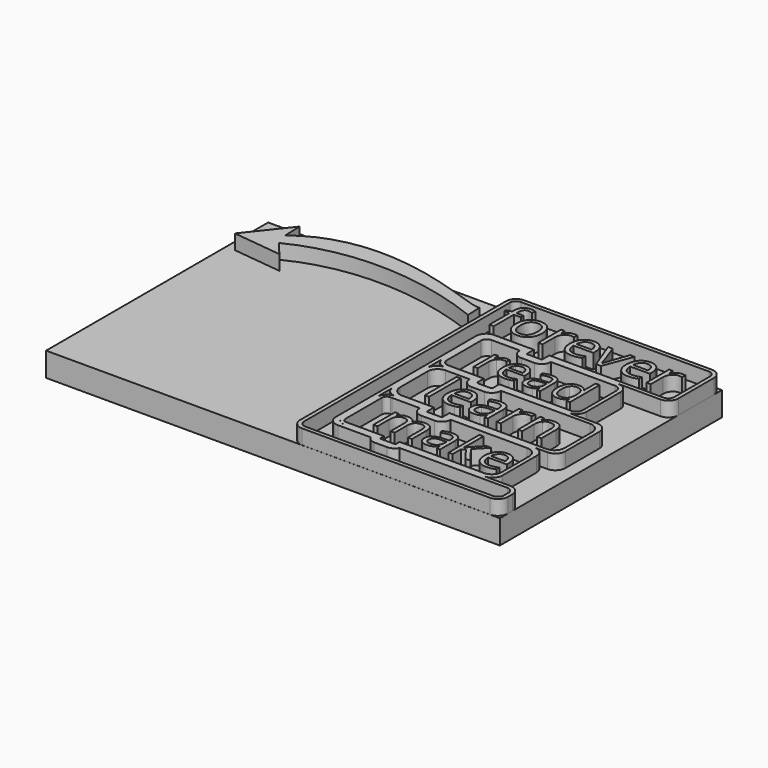
from build123d import *

# Parameters (mm, degrees)
F0_TEXT_SIZE   = 5.4091811762
F0_W           = 0.4318574544
F0_H           = 4.046479385
F1_DEPTH       = 1.5
F0_TEXT_SIZE_2 = 5.1478958792
F2_DEPTH       = 1.5
F3_DEPTH       = 1.5
F4_DEPTH       = 1.5
F5_W           = 28.2222777605
F5_H           = 2.4435883388
F6_DEPTH       = 21.1379435506
F7_DEPTH       = 25
F9_DEPTH       = 1.5


# Not quite as in the source:
# - ends of sketch curves that miss each other by under 0.0002 mm in the source are joined
# - Text() gives the source's letters only with a copy of the font that has no kerning and outlines rounded to 1/6400 em; it was checked with that copy


with BuildPart() as f1:
    # F0 (on Top) → F1 (new body)
    with BuildSketch(Plane.XY):
        with Locations((-20.2342048287, -5.0012101419)):
            Text('forever', F0_TEXT_SIZE, font='Open Sans', text_align=(TextAlign.LEFT, TextAlign.BOTTOM))
        with BuildLine():
            add(Edge.make_bspline(
                [(-14.8840140161, -8.7097081899), (-14.7069441142, -8.7097081899), (-14.5663754641, -8.7392198402)],
                knots=[0, 0, 0, 1, 1, 1], degree=2))
            add(Edge.make_bspline(
                [(-15.3429978406, -8.8506651512), (-15.1340864213, -8.7097081899), (-14.8840140161, -8.7097081899)],
                knots=[0, 0, 0, 1, 1, 1], degree=2))
            add(Edge.make_bspline(
                [(-15.6994675114, -9.2510139863), (-15.5519092599, -8.9916221126), (-15.3429978406, -8.8506651512)],
                knots=[0, 0, 0, 1, 1, 1], degree=2))
            Line((-15.6994675114, -9.2510139863), (-15.7188830708, -9.2510139863))
            Line((-15.7188830708, -9.2510139863), (-15.7654804134, -8.7586353996))
            Line((-15.7654804134, -8.7586353996), (-16.0978747905, -8.7586353996))
            Line((-16.0978747905, -8.7586353996), (-16.0978747905, -11.4185670391))
            Line((-16.0978747905, -11.4185670391), (-15.6948077771, -11.4185670391))
            Line((-15.6948077771, -11.4185670391), (-15.6948077771, -9.9911351111))
            add(Edge.make_bspline(
                [(-15.4657041761, -9.3383840037), (-15.6948077771, -9.6004940557), (-15.6948077771, -9.9911351111)],
                knots=[0, 0, 0, 1, 1, 1], degree=2))
            add(Edge.make_bspline(
                [(-14.9135256664, -9.0762739516), (-15.236600575, -9.0762739516), (-15.4657041761, -9.3383840037)],
                knots=[0, 0, 0, 1, 1, 1], degree=2))
            add(Edge.make_bspline(
                [(-14.6222922752, -9.1127752033), (-14.786936219, -9.0762739516), (-14.9135256664, -9.0762739516)],
                knots=[0, 0, 0, 1, 1, 1], degree=2))
            Line((-14.6222922752, -9.1127752033), (-14.5663754641, -8.7392198402))
        make_face()
        with BuildLine():
            add(Edge.make_bspline(
                [(-12.944787942, -11.4674942488), (-13.5342443258, -11.4674942488), (-13.8755698602, -11.1079180885)],
                knots=[0, 0, 0, 1, 1, 1], degree=2))
            add(Edge.make_bspline(
                [(-12.4850274951, -11.4271098852), (-12.6752999774, -11.4674942488), (-12.944787942, -11.4674942488)],
                knots=[0, 0, 0, 1, 1, 1], degree=2))
            add(Edge.make_bspline(
                [(-12.0811838594, -11.2950840812), (-12.2947550129, -11.3867255216), (-12.4850274951, -11.4271098852)],
                knots=[0, 0, 0, 1, 1, 1], degree=2))
            Line((-12.0811838594, -11.2950840812), (-12.0811838594, -10.9355079209))
            add(Edge.make_bspline(
                [(-12.9300321169, -11.1149076899), (-12.5005599427, -11.1149076899), (-12.0811838594, -10.9355079209)],
                knots=[0, 0, 0, 1, 1, 1], degree=2))
            add(Edge.make_bspline(
                [(-13.5622027313, -10.8722131972), (-13.3377588645, -11.1149076899), (-12.9300321169, -11.1149076899)],
                knots=[0, 0, 0, 1, 1, 1], degree=2))
            add(Edge.make_bspline(
                [(-13.7990725561, -10.1612154115), (-13.7866465981, -10.6295187046), (-13.5622027313, -10.8722131972)],
                knots=[0, 0, 0, 1, 1, 1], degree=2))
            Line((-13.7990725561, -10.1612154115), (-11.96702037, -10.1612154115))
            Line((-11.96702037, -10.1612154115), (-11.96702037, -9.9064832721))
            add(Edge.make_bspline(
                [(-12.2582537612, -9.0386077663), (-11.96702037, -9.3675073428), (-11.96702037, -9.9064832721)],
                knots=[0, 0, 0, 1, 1, 1], degree=2))
            add(Edge.make_bspline(
                [(-13.0488553405, -8.7097081899), (-12.5494871524, -8.7097081899), (-12.2582537612, -9.0386077663)],
                knots=[0, 0, 0, 1, 1, 1], degree=2))
            add(Edge.make_bspline(
                [(-13.9000334651, -9.0883115984), (-13.5831715355, -8.7097081899), (-13.0488553405, -8.7097081899)],
                knots=[0, 0, 0, 1, 1, 1], degree=2))
            add(Edge.make_bspline(
                [(-14.2168953947, -10.1107349571), (-14.2168953947, -9.466915007), (-13.9000334651, -9.0883115984)],
                knots=[0, 0, 0, 1, 1, 1], degree=2))
            add(Edge.make_bspline(
                [(-13.8755698602, -11.1079180885), (-14.2168953947, -10.7483419282), (-14.2168953947, -10.1107349571)],
                knots=[0, 0, 0, 1, 1, 1], degree=2))
        make_face()
        with BuildLine():
            add(Edge.make_bspline(
                [(-13.0542916971, -9.0475389237), (-13.3742601162, -9.0475389237), (-13.5649209096, -9.2560620318)],
                knots=[0, 0, 0, 1, 1, 1], degree=2))
            add(Edge.make_bspline(
                [(-12.5685144006, -9.2502373639), (-12.7382063899, -9.0475389237), (-13.0542916971, -9.0475389237)],
                knots=[0, 0, 0, 1, 1, 1], degree=2))
            add(Edge.make_bspline(
                [(-12.3988224113, -9.8334807687), (-12.3988224113, -9.4529358042), (-12.5685144006, -9.2502373639)],
                knots=[0, 0, 0, 1, 1, 1], degree=2))
            Line((-12.3988224113, -9.8334807687), (-13.7897530876, -9.8334807687))
            add(Edge.make_bspline(
                [(-13.5649209096, -9.2560620318), (-13.7555817031, -9.4645851398), (-13.7897530876, -9.8334807687)],
                knots=[0, 0, 0, 1, 1, 1], degree=2))
        make_face(mode=Mode.SUBTRACT)
        with BuildLine():
            Line((-9.7241349467, -11.0395753193), (-9.644142842, -11.4185670391))
            Line((-9.644142842, -11.4185670391), (-9.345143227, -11.4185670391))
            Line((-9.345143227, -11.4185670391), (-9.345143227, -9.6028239229))
            add(Edge.make_bspline(
                [(-9.5746351393, -8.9259975218), (-9.345143227, -9.136850497), (-9.345143227, -9.6028239229)],
                knots=[0, 0, 0, 1, 1, 1], degree=2))
            add(Edge.make_bspline(
                [(-10.2794199459, -8.7151445465), (-9.8041270515, -8.7151445465), (-9.5746351393, -8.9259975218)],
                knots=[0, 0, 0, 1, 1, 1], degree=2))
            add(Edge.make_bspline(
                [(-10.7496647949, -8.7757210919), (-10.5155131484, -8.7151445465), (-10.2794199459, -8.7151445465)],
                knots=[0, 0, 0, 1, 1, 1], degree=2))
            add(Edge.make_bspline(
                [(-11.1803019026, -8.9426949028), (-10.9838164414, -8.8362976373), (-10.7496647949, -8.7757210919)],
                knots=[0, 0, 0, 1, 1, 1], degree=2))
            Line((-11.1803019026, -8.9426949028), (-11.0560423224, -9.2510139863))
            add(Edge.make_bspline(
                [(-10.304271862, -9.0475389237), (-10.6366662391, -9.0475389237), (-11.0560423224, -9.2510139863)],
                knots=[0, 0, 0, 1, 1, 1], degree=2))
            add(Edge.make_bspline(
                [(-9.873246443, -9.19665042), (-10.0076021142, -9.0475389237), (-10.304271862, -9.0475389237)],
                knots=[0, 0, 0, 1, 1, 1], degree=2))
            add(Edge.make_bspline(
                [(-9.7388907719, -9.658740734), (-9.7388907719, -9.3457619162), (-9.873246443, -9.19665042)],
                knots=[0, 0, 0, 1, 1, 1], degree=2))
            Line((-9.7388907719, -9.658740734), (-9.7388907719, -9.8241613002))
            Line((-9.7388907719, -9.8241613002), (-10.1901083726, -9.8389171253))
            add(Edge.make_bspline(
                [(-11.4785248952, -10.6831056485), (-11.4785248952, -9.8777482441), (-10.1901083726, -9.8389171253)],
                knots=[0, 0, 0, 1, 1, 1], degree=2))
            add(Edge.make_bspline(
                [(-11.2540810284, -11.2632425638), (-11.4785248952, -11.0589908788), (-11.4785248952, -10.6831056485)],
                knots=[0, 0, 0, 1, 1, 1], degree=2))
            add(Edge.make_bspline(
                [(-10.634336372, -11.4674942488), (-11.0296371616, -11.4674942488), (-11.2540810284, -11.2632425638)],
                knots=[0, 0, 0, 1, 1, 1], degree=2))
            add(Edge.make_bspline(
                [(-10.1400162293, -11.3785709867), (-10.3376666242, -11.4674942488), (-10.634336372, -11.4674942488)],
                knots=[0, 0, 0, 1, 1, 1], degree=2))
            add(Edge.make_bspline(
                [(-9.7435505061, -11.0395753193), (-9.9423658345, -11.2896477246), (-10.1400162293, -11.3785709867)],
                knots=[0, 0, 0, 1, 1, 1], degree=2))
            Line((-9.7435505061, -11.0395753193), (-9.7241349467, -11.0395753193))
        make_face()
        with BuildLine():
            add(Edge.make_bspline(
                [(-10.5543442672, -11.1343232493), (-10.1776824146, -11.1343232493), (-9.9629463275, -10.9281300083)],
                knots=[0, 0, 0, 1, 1, 1], degree=2))
            add(Edge.make_bspline(
                [(-10.9240165184, -11.0205480711), (-10.7919907144, -11.1343232493), (-10.5543442672, -11.1343232493)],
                knots=[0, 0, 0, 1, 1, 1], degree=2))
            add(Edge.make_bspline(
                [(-11.0560423224, -10.6877653828), (-11.0560423224, -10.906772893), (-10.9240165184, -11.0205480711)],
                knots=[0, 0, 0, 1, 1, 1], degree=2))
            add(Edge.make_bspline(
                [(-10.8440244136, -10.2765438345), (-11.0560423224, -10.4089579496), (-11.0560423224, -10.6877653828)],
                knots=[0, 0, 0, 1, 1, 1], degree=2))
            add(Edge.make_bspline(
                [(-10.1512772538, -10.127044027), (-10.6320065048, -10.1441297193), (-10.8440244136, -10.2765438345)],
                knots=[0, 0, 0, 1, 1, 1], degree=2))
            Line((-10.1512772538, -10.127044027), (-9.7482102404, -10.1107349571))
            Line((-9.7482102404, -10.1107349571), (-9.7482102404, -10.3507112714))
            add(Edge.make_bspline(
                [(-9.9629463275, -10.9281300083), (-9.7482102404, -10.7219367674), (-9.7482102404, -10.3507112714)],
                knots=[0, 0, 0, 1, 1, 1], degree=2))
        make_face(mode=Mode.SUBTRACT)
        with Locations((-15.8514359621, -15.6580106562)):
            Rectangle(F0_W, F0_H)
    extrude(amount=F1_DEPTH)


with BuildPart() as f2:
    # F0 (on Top) → F2 (new body)
    with BuildSketch(Plane.XY):
        with Locations((-16.5250170976, -24.199552834)):
            Text('make', F0_TEXT_SIZE_2, font='Open Sans', text_align=(TextAlign.LEFT, TextAlign.BOTTOM))
    extrude(amount=F2_DEPTH)


with BuildPart() as f3:
    # F0 (on Top) → F3 (new body)
    with BuildSketch(Plane.XY):
        with BuildLine():
            add(Edge.make_bspline(
                [(-13.5161605366, -17.7336723518), (-14.1477208601, -17.7336723518), (-14.5134267391, -17.3484122335)],
                knots=[0, 0, 0, 1, 1, 1], degree=2))
            add(Edge.make_bspline(
                [(-13.0235601262, -17.6904033969), (-13.2274234717, -17.7336723518), (-13.5161605366, -17.7336723518)],
                knots=[0, 0, 0, 1, 1, 1], degree=2))
            add(Edge.make_bspline(
                [(-12.5908705765, -17.5489471979), (-12.8196967807, -17.6471344419), (-13.0235601262, -17.6904033969)],
                knots=[0, 0, 0, 1, 1, 1], degree=2))
            Line((-12.5908705765, -17.5489471979), (-12.5908705765, -17.1636870796))
            add(Edge.make_bspline(
                [(-13.5003507261, -17.3559010911), (-13.0402020319, -17.3559010911), (-12.5908705765, -17.1636870796)],
                knots=[0, 0, 0, 1, 1, 1], degree=2))
            add(Edge.make_bspline(
                [(-14.1776762905, -17.0958713137), (-13.9372007523, -17.3559010911), (-13.5003507261, -17.3559010911)],
                knots=[0, 0, 0, 1, 1, 1], degree=2))
            add(Edge.make_bspline(
                [(-14.4314653533, -16.3340880776), (-14.4181518287, -16.8358415362), (-14.1776762905, -17.0958713137)],
                knots=[0, 0, 0, 1, 1, 1], degree=2))
            Line((-14.4314653533, -16.3340880776), (-12.4685525692, -16.3340880776))
            Line((-12.4685525692, -16.3340880776), (-12.4685525692, -16.0611608232))
            add(Edge.make_bspline(
                [(-12.7805883021, -15.131294339), (-12.4685525692, -15.4836866934), (-12.4685525692, -16.0611608232)],
                knots=[0, 0, 0, 1, 1, 1], degree=2))
            add(Edge.make_bspline(
                [(-13.6276613052, -14.7789019846), (-13.0926240351, -14.7789019846), (-12.7805883021, -15.131294339)],
                knots=[0, 0, 0, 1, 1, 1], degree=2))
            add(Edge.make_bspline(
                [(-14.5396377407, -15.1845484374), (-14.2001428632, -14.7789019846), (-13.6276613052, -14.7789019846)],
                knots=[0, 0, 0, 1, 1, 1], degree=2))
            add(Edge.make_bspline(
                [(-14.8791326182, -16.2800018839), (-14.8791326182, -15.5901948902), (-14.5396377407, -15.1845484374)],
                knots=[0, 0, 0, 1, 1, 1], degree=2))
            add(Edge.make_bspline(
                [(-14.5134267391, -17.3484122335), (-14.8791326182, -16.9631521152), (-14.8791326182, -16.2800018839)],
                knots=[0, 0, 0, 1, 1, 1], degree=2))
        make_face()
        with BuildLine():
            add(Edge.make_bspline(
                [(-13.6334859722, -15.1408634348), (-13.9763092308, -15.1408634348), (-14.180588624, -15.3642810196)],
                knots=[0, 0, 0, 1, 1, 1], degree=2))
            add(Edge.make_bspline(
                [(-13.1130103696, -15.3580403049), (-13.29482319, -15.1408634348), (-13.6334859722, -15.1408634348)],
                knots=[0, 0, 0, 1, 1, 1], degree=2))
            add(Edge.make_bspline(
                [(-12.9311975492, -15.9829438661), (-12.9311975492, -15.5752171751), (-13.1130103696, -15.3580403049)],
                knots=[0, 0, 0, 1, 1, 1], degree=2))
            Line((-12.9311975492, -15.9829438661), (-14.4214802098, -15.9829438661))
            add(Edge.make_bspline(
                [(-14.180588624, -15.3642810196), (-14.3848680172, -15.5876986044), (-14.4214802098, -15.9829438661)],
                knots=[0, 0, 0, 1, 1, 1], degree=2))
        make_face(mode=Mode.SUBTRACT)
        with BuildLine():
            Line((-10.0654613778, -17.2751878482), (-9.9797555631, -17.6812503487))
            Line((-9.9797555631, -17.6812503487), (-9.6593988773, -17.6812503487))
            Line((-9.6593988773, -17.6812503487), (-9.6593988773, -15.7358115656))
            add(Edge.make_bspline(
                [(-9.9052830348, -15.0106405222), (-9.6593988773, -15.2365543929), (-9.6593988773, -15.7358115656)],
                knots=[0, 0, 0, 1, 1, 1], degree=2))
            add(Edge.make_bspline(
                [(-10.6604095086, -14.7847266516), (-10.1511671924, -14.7847266516), (-9.9052830348, -15.0106405222)],
                knots=[0, 0, 0, 1, 1, 1], degree=2))
            add(Edge.make_bspline(
                [(-11.1642432054, -14.849630084), (-10.9133664761, -14.7847266516), (-10.6604095086, -14.7847266516)],
                knots=[0, 0, 0, 1, 1, 1], degree=2))
            add(Edge.make_bspline(
                [(-11.6256400425, -15.0285305709), (-11.4151199347, -14.9145335165), (-11.1642432054, -14.849630084)],
                knots=[0, 0, 0, 1, 1, 1], degree=2))
            Line((-11.6256400425, -15.0285305709), (-11.4925047965, -15.3588724002))
            add(Edge.make_bspline(
                [(-10.6870365578, -15.1408634348), (-11.043173341, -15.1408634348), (-11.4925047965, -15.3588724002)],
                knots=[0, 0, 0, 1, 1, 1], degree=2))
            add(Edge.make_bspline(
                [(-10.225223673, -15.3006257301), (-10.3691761578, -15.1408634348), (-10.6870365578, -15.1408634348)],
                knots=[0, 0, 0, 1, 1, 1], degree=2))
            add(Edge.make_bspline(
                [(-10.0812711882, -15.7957224263), (-10.0812711882, -15.4603880253), (-10.225223673, -15.3006257301)],
                knots=[0, 0, 0, 1, 1, 1], degree=2))
            Line((-10.0812711882, -15.7957224263), (-10.0812711882, -15.9729587227))
            Line((-10.0812711882, -15.9729587227), (-10.5647185505, -15.9887685331))
            add(Edge.make_bspline(
                [(-11.9451646331, -16.8932561111), (-11.9451646331, -16.0303732975), (-10.5647185505, -15.9887685331)],
                knots=[0, 0, 0, 1, 1, 1], degree=2))
            add(Edge.make_bspline(
                [(-11.7046890949, -17.5148312911), (-11.9451646331, -17.2959902304), (-11.9451646331, -16.8932561111)],
                knots=[0, 0, 0, 1, 1, 1], degree=2))
            add(Edge.make_bspline(
                [(-11.0406770552, -17.7336723518), (-11.4642135567, -17.7336723518), (-11.7046890949, -17.5148312911)],
                knots=[0, 0, 0, 1, 1, 1], degree=2))
            add(Edge.make_bspline(
                [(-10.5110484044, -17.6383974414), (-10.7228166552, -17.7336723518), (-11.0406770552, -17.7336723518)],
                knots=[0, 0, 0, 1, 1, 1], degree=2))
            add(Edge.make_bspline(
                [(-10.08626376, -17.2751878482), (-10.2992801537, -17.5431225309), (-10.5110484044, -17.6383974414)],
                knots=[0, 0, 0, 1, 1, 1], degree=2))
            Line((-10.08626376, -17.2751878482), (-10.0654613778, -17.2751878482))
        make_face()
        with BuildLine():
            add(Edge.make_bspline(
                [(-10.9549712405, -17.3767034733), (-10.5514050259, -17.3767034733), (-10.3213306788, -17.1557821744)],
                knots=[0, 0, 0, 1, 1, 1], degree=2))
            add(Edge.make_bspline(
                [(-11.3510485975, -17.2548015136), (-11.2095923986, -17.3767034733), (-10.9549712405, -17.3767034733)],
                knots=[0, 0, 0, 1, 1, 1], degree=2))
            add(Edge.make_bspline(
                [(-11.4925047965, -16.8982486828), (-11.4925047965, -17.132899554), (-11.3510485975, -17.2548015136)],
                knots=[0, 0, 0, 1, 1, 1], degree=2))
            add(Edge.make_bspline(
                [(-11.2653427829, -16.4576542279), (-11.4925047965, -16.5995264744), (-11.4925047965, -16.8982486828)],
                knots=[0, 0, 0, 1, 1, 1], degree=2))
            add(Edge.make_bspline(
                [(-10.5231137861, -16.2974758849), (-11.0381807693, -16.3157819813), (-11.2653427829, -16.4576542279)],
                knots=[0, 0, 0, 1, 1, 1], degree=2))
            Line((-10.5231137861, -16.2974758849), (-10.0912563317, -16.2800018839))
            Line((-10.0912563317, -16.2800018839), (-10.0912563317, -16.5371193278))
            add(Edge.make_bspline(
                [(-10.3213306788, -17.1557821744), (-10.0912563317, -16.9348608755), (-10.0912563317, -16.5371193278)],
                knots=[0, 0, 0, 1, 1, 1], degree=2))
        make_face(mode=Mode.SUBTRACT)
        with BuildLine():
            add(Edge.make_bspline(
                [(-7.4701561749, -14.7789019846), (-7.2804384492, -14.7789019846), (-7.1298292021, -14.8105216055)],
                knots=[0, 0, 0, 1, 1, 1], degree=2))
            add(Edge.make_bspline(
                [(-7.96192449, -14.9299272793), (-7.7380908576, -14.7789019846), (-7.4701561749, -14.7789019846)],
                knots=[0, 0, 0, 1, 1, 1], degree=2))
            add(Edge.make_bspline(
                [(-8.3438562271, -15.3588724002), (-8.1857581224, -15.0809525741), (-7.96192449, -14.9299272793)],
                knots=[0, 0, 0, 1, 1, 1], degree=2))
            Line((-8.3438562271, -15.3588724002), (-8.3646586093, -15.3588724002))
            Line((-8.3646586093, -15.3588724002), (-8.4145843266, -14.8313239877))
            Line((-8.4145843266, -14.8313239877), (-8.7707211098, -14.8313239877))
            Line((-8.7707211098, -14.8313239877), (-8.7707211098, -17.6812503487))
            Line((-8.7707211098, -17.6812503487), (-8.3388636554, -17.6812503487))
            Line((-8.3388636554, -17.6812503487), (-8.3388636554, -16.1518592096))
            add(Edge.make_bspline(
                [(-8.0933955455, -15.4524831201), (-8.3388636554, -15.7333152798), (-8.3388636554, -16.1518592096)],
                knots=[0, 0, 0, 1, 1, 1], degree=2))
            add(Edge.make_bspline(
                [(-7.5017757958, -15.1716509604), (-7.8479274356, -15.1716509604), (-8.0933955455, -15.4524831201)],
                knots=[0, 0, 0, 1, 1, 1], degree=2))
            add(Edge.make_bspline(
                [(-7.1897400628, -15.210759439), (-7.3661442639, -15.1716509604), (-7.5017757958, -15.1716509604)],
                knots=[0, 0, 0, 1, 1, 1], degree=2))
            Line((-7.1897400628, -15.210759439), (-7.1298292021, -14.8105216055))
        make_face()
        with BuildLine():
            Line((-4.6460247678, -15.8373271907), (-4.6460247678, -17.6812503487))
            Line((-4.6460247678, -17.6812503487), (-4.2141673134, -17.6812503487))
            Line((-4.2141673134, -17.6812503487), (-4.2141673134, -15.8223494756))
            add(Edge.make_bspline(
                [(-4.4741970908, -15.027282428), (-4.2141673134, -15.2756628714), (-4.2141673134, -15.8223494756)],
                knots=[0, 0, 0, 1, 1, 1], degree=2))
            add(Edge.make_bspline(
                [(-5.2492938515, -14.7789019846), (-4.7342268683, -14.7789019846), (-4.4741970908, -15.027282428)],
                knots=[0, 0, 0, 1, 1, 1], degree=2))
            add(Edge.make_bspline(
                [(-5.7822508834, -14.8949792772), (-5.5430234881, -14.7789019846), (-5.2492938515, -14.7789019846)],
                knots=[0, 0, 0, 1, 1, 1], degree=2))
            add(Edge.make_bspline(
                [(-6.1546135247, -15.2215766777), (-6.0214782787, -15.0110565699), (-5.7822508834, -14.8949792772)],
                knots=[0, 0, 0, 1, 1, 1], degree=2))
            Line((-6.1546135247, -15.2215766777), (-6.1754159069, -15.2215766777))
            Line((-6.1754159069, -15.2215766777), (-6.2453119111, -14.8313239877))
            Line((-6.2453119111, -14.8313239877), (-6.5964561226, -14.8313239877))
            Line((-6.5964561226, -14.8313239877), (-6.5964561226, -17.6812503487))
            Line((-6.5964561226, -17.6812503487), (-6.1645986682, -17.6812503487))
            Line((-6.1645986682, -17.6812503487), (-6.1645986682, -16.1859751164))
            add(Edge.make_bspline(
                [(-5.9565748462, -15.3875796876), (-6.1645986682, -15.6293033688), (-6.1645986682, -16.1859751164)],
                knots=[0, 0, 0, 1, 1, 1], degree=2))
            add(Edge.make_bspline(
                [(-5.3017158546, -15.1458560065), (-5.7485510242, -15.1458560065), (-5.9565748462, -15.3875796876)],
                knots=[0, 0, 0, 1, 1, 1], degree=2))
            add(Edge.make_bspline(
                [(-4.8045389201, -15.3176836835), (-4.9630530725, -15.1458560065), (-5.3017158546, -15.1458560065)],
                knots=[0, 0, 0, 1, 1, 1], degree=2))
            add(Edge.make_bspline(
                [(-4.6460247678, -15.8373271907), (-4.6460247678, -15.4895113604), (-4.8045389201, -15.3176836835)],
                knots=[0, 0, 0, 1, 1, 1], degree=2))
        make_face()
    extrude(amount=F3_DEPTH)


with BuildPart() as f4:
    # F0 (on Top) → F4 (new body)
    with BuildSketch(Plane.XY):
        with BuildLine():
            ThreePointArc((0, -1.016), (-0.2975795103, -0.2975795103), (-1.016, 0))
            Line((-1.016, 0), (-20.1219435506, 0))
            ThreePointArc((-20.1219435506, 0), (-20.8403640403, -0.2975795103), (-21.1379435506, -1.016))
            Line((-21.1379435506, -1.016), (-21.1379435506, -27.1978804077))
            ThreePointArc((-21.1379435506, -27.1978804077), (-20.8403640403, -27.9163008974), (-20.1219435506, -28.2138804077))
            Line((-20.1219435506, -28.2138804077), (-1.016, -28.2138804077))
            ThreePointArc((-1.016, -28.2138804077), (-0.2975795103, -27.9163008974), (0, -27.1978804077))
            Line((0, -27.1978804077), (0, -26.6231552621))
            ThreePointArc((0, -26.6231552621), (-0.2975795103, -25.9047347724), (-1.016, -25.6071552621))
            Line((-1.016, -25.6071552621), (-3.6488115588, -25.6071552621))
            Line((-3.6488115588, -25.6071552621), (-4.0488115588, -25.6071552621))
            Line((-4.0488115588, -25.6071552621), (-11.8191120928, -25.6071552621))
            Line((-11.8191120928, -25.6071552621), (-11.8242466355, -25.6071552621))
            Line((-11.8242466355, -25.6071552621), (-12.2191120928, -25.6071552621))
            Line((-12.2191120928, -25.6071552621), (-12.2191120928, -25.6131404206))
            ThreePointArc((-12.2191120928, -25.6131404206), (-12.3679018479, -25.9723506654), (-12.7271120928, -26.1211404206))
            Line((-12.7271120928, -26.1211404206), (-14.0753652451, -26.1211404206))
            ThreePointArc((-14.0753652451, -26.1211404206), (-14.43457549, -25.9723506654), (-14.5833652451, -25.6131404206))
            Line((-14.5833652451, -25.6131404206), (-14.5833652451, -25.6071552621))
            Line((-14.5833652451, -25.6071552621), (-14.9833652451, -25.6071552621))
            Line((-14.9833652451, -25.6071552621), (-17.8403063085, -25.6071552621))
            Line((-17.8403063085, -25.6071552621), (-17.8563063085, -25.6071552621))
            ThreePointArc((-17.8563063085, -25.6071552621), (-18.5634130897, -25.3142620433), (-18.8563063085, -24.6071552621))
            Line((-18.8563063085, -24.6071552621), (-18.8563063085, -24.5911552621))
            Line((-18.8563063085, -24.5911552621), (-18.8563063085, -20.2731552621))
            Line((-18.8563063085, -20.2731552621), (-18.8563063085, -19.2571552621))
            Line((-18.8563063085, -19.2571552621), (-18.8563063085, -18.2411552621))
            Line((-18.8563063085, -18.2411552621), (-18.8563063085, -13.9231552621))
            Line((-18.8563063085, -13.9231552621), (-18.8563063085, -11.8911552621))
            Line((-18.8563063085, -11.8911552621), (-18.8563063085, -7.5731552621))
            ThreePointArc((-18.8563063085, -7.5731552621), (-18.5587267982, -6.8547347724), (-17.8403063085, -6.5571552621))
            Line((-17.8403063085, -6.5571552621), (-14.5908056537, -6.5571552621))
            Line((-14.5908056537, -6.5571552621), (-14.5908056537, -6.9889552621))
            ThreePointArc((-14.5908056537, -6.9889552621), (-14.4420158986, -7.348165507), (-14.0828056537, -7.4969552621))
            Line((-14.0828056537, -7.4969552621), (-12.7345525014, -7.4969552621))
            ThreePointArc((-12.7345525014, -7.4969552621), (-12.3753422565, -7.348165507), (-12.2265525014, -6.9889552621))
            Line((-12.2265525014, -6.9889552621), (-12.2265525014, -6.5571552621))
            Line((-12.2265525014, -6.5571552621), (-5.2834429959, -6.5571552621))
            Line((-5.2834429959, -6.5571552621), (-1.016, -6.5571552621))
            ThreePointArc((-1.016, -6.5571552621), (-0.2975795103, -6.2595757518), (0, -5.5411552621))
            Line((0, -5.5411552621), (0, -1.016))
        make_face()
        with BuildLine():
            Line((-20.1219435506, -0.4), (-1.016, -0.4))
            ThreePointArc((-1.016, -0.4), (-0.5804222228, -0.5804222228), (-0.4, -1.016))
            Line((-0.4, -1.016), (-0.4, -5.5411552621))
            ThreePointArc((-0.4, -5.5411552621), (-0.5804222228, -5.9767330393), (-1.016, -6.1571552621))
            Line((-1.016, -6.1571552621), (-12.2265525014, -6.1571552621))
            Line((-12.2265525014, -6.1571552621), (-12.6265525014, -6.1571552621))
            Line((-12.6265525014, -6.1571552621), (-12.6265525014, -7.0344238815))
            ThreePointArc((-12.6265525014, -7.0344238815), (-12.6448675187, -7.0786402448), (-12.689083882, -7.0969552621))
            Line((-12.689083882, -7.0969552621), (-14.0828056537, -7.0969552621))
            Line((-14.0828056537, -7.0969552621), (-14.1282742731, -7.0969552621))
            ThreePointArc((-14.1282742731, -7.0969552621), (-14.1724906364, -7.0786402448), (-14.1908056537, -7.0344238815))
            Line((-14.1908056537, -7.0344238815), (-14.1908056537, -6.1571552621))
            Line((-14.1908056537, -6.1571552621), (-18.2403063085, -6.1571552621))
            ThreePointArc((-18.2403063085, -6.1571552621), (-18.9587267982, -6.4547347724), (-19.2563063085, -7.1731552621))
            Line((-19.2563063085, -7.1731552621), (-19.2563063085, -24.5911552621))
            Line((-19.2563063085, -24.5911552621), (-19.2563063085, -24.9911552621))
            ThreePointArc((-19.2563063085, -24.9911552621), (-18.9587267982, -25.7095757518), (-18.2403063085, -26.0071552621))
            Line((-18.2403063085, -26.0071552621), (-17.8403063085, -26.0071552621))
            Line((-17.8403063085, -26.0071552621), (-14.898319214, -26.0071552621))
            ThreePointArc((-14.898319214, -26.0071552621), (-14.6014851036, -26.3610162099), (-14.1682550311, -26.5211404234))
            Line((-14.1682550311, -26.5211404234), (-12.8351120928, -26.5211404234))
            ThreePointArc((-12.8351120928, -26.5211404234), (-12.3241282751, -26.3832927667), (-11.9518017839, -26.0071552621))
            Line((-11.9518017839, -26.0071552621), (-1.016, -26.0071552621))
            ThreePointArc((-1.016, -26.0071552621), (-0.5804222228, -26.1875774849), (-0.4, -26.6231552621))
            Line((-0.4, -26.6231552621), (-0.4, -27.1978804077))
            ThreePointArc((-0.4, -27.1978804077), (-0.5804222228, -27.6334581849), (-1.016, -27.8138804077))
            Line((-1.016, -27.8138804077), (-20.1219435506, -27.8138804077))
            ThreePointArc((-20.1219435506, -27.8138804077), (-20.5575213278, -27.6334581849), (-20.7379435506, -27.1978804077))
            Line((-20.7379435506, -27.1978804077), (-20.7379435506, -1.016))
            ThreePointArc((-20.7379435506, -1.016), (-20.5575213278, -0.5804222228), (-20.1219435506, -0.4))
        make_face(mode=Mode.SUBTRACT)
        with BuildLine():
            Line((-2.3438170035, -12.9071552621), (-5.2834429959, -12.9071552621))
            Line((-5.2834429959, -12.9071552621), (-12.2265525014, -12.9071552621))
            Line((-12.2265525014, -12.9071552621), (-12.2265525014, -13.3389552621))
            ThreePointArc((-12.2265525014, -13.3389552621), (-12.3753422565, -13.698165507), (-12.7345525014, -13.8469552621))
            Line((-12.7345525014, -13.8469552621), (-14.0828056537, -13.8469552621))
            ThreePointArc((-14.0828056537, -13.8469552621), (-14.4420158986, -13.698165507), (-14.5908056537, -13.3389552621))
            Line((-14.5908056537, -13.3389552621), (-14.5908056537, -12.9071552621))
            Line((-14.5908056537, -12.9071552621), (-17.8403063085, -12.9071552621))
            ThreePointArc((-17.8403063085, -12.9071552621), (-18.5587267982, -13.2047347724), (-18.8563063085, -13.9231552621))
            Line((-18.8563063085, -13.9231552621), (-18.8563063085, -18.2411552621))
            ThreePointArc((-18.8563063085, -18.2411552621), (-18.5587267982, -18.9595757518), (-17.8403063085, -19.2571552621))
            Line((-17.8403063085, -19.2571552621), (-14.5908056537, -19.2571552621))
            Line((-14.5908056537, -19.2571552621), (-14.5908056537, -19.6889552621))
            ThreePointArc((-14.5908056537, -19.6889552621), (-14.4420158986, -20.048165507), (-14.0828056537, -20.1969552621))
            Line((-14.0828056537, -20.1969552621), (-12.7345525014, -20.1969552621))
            ThreePointArc((-12.7345525014, -20.1969552621), (-12.3753422565, -20.048165507), (-12.2265525014, -19.6889552621))
            Line((-12.2265525014, -19.6889552621), (-12.2265525014, -19.2571552621))
            Line((-12.2265525014, -19.2571552621), (-4.0488115588, -19.2571552621))
            Line((-4.0488115588, -19.2571552621), (-3.6488115588, -19.2571552621))
            Line((-3.6488115588, -19.2571552621), (-2.3438170035, -19.2571552621))
            ThreePointArc((-2.3438170035, -19.2571552621), (-1.6253965138, -18.9595757518), (-1.3278170035, -18.2411552621))
            Line((-1.3278170035, -18.2411552621), (-1.3278170035, -13.9231552621))
            ThreePointArc((-1.3278170035, -13.9231552621), (-1.6253965138, -13.2047347724), (-2.3438170035, -12.9071552621))
        make_face()
        with BuildLine():
            Line((-18.4563063085, -17.8411552621), (-18.4563063085, -14.7484978661))
            Line((-18.4563063085, -14.7484978661), (-18.4563063085, -14.3231552621))
            ThreePointArc((-18.4563063085, -14.3231552621), (-18.1587267982, -13.6047347724), (-17.4403063085, -13.3071552621))
            Line((-17.4403063085, -13.3071552621), (-14.9902486326, -13.3071552621))
            ThreePointArc((-14.9902486326, -13.3071552621), (-14.7360048576, -13.969665021), (-14.0828056537, -14.2469552621))
            Line((-14.0828056537, -14.2469552621), (-12.7345525014, -14.2469552621))
            ThreePointArc((-12.7345525014, -14.2469552621), (-12.0813532975, -13.969665021), (-11.8271095225, -13.3071552621))
            Line((-11.8271095225, -13.3071552621), (-2.7438170035, -13.3071552621))
            ThreePointArc((-2.7438170035, -13.3071552621), (-2.0253965138, -13.6047347724), (-1.7278170035, -14.3231552621))
            Line((-1.7278170035, -14.3231552621), (-1.7278170035, -15.827415511))
            Line((-1.7278170035, -15.827415511), (-1.7278170035, -17.840364294))
            ThreePointArc((-1.7278170035, -17.840364294), (-2.0253665523, -18.558754821), (-2.7437322579, -18.8563642905))
            Line((-2.7437322579, -18.8563642905), (-12.2265525014, -18.8571552621))
            Line((-12.2265525014, -18.8571552621), (-12.6265525014, -18.8571552621))
            Line((-12.6265525014, -18.8571552621), (-12.6265525014, -19.2571552621))
            Line((-12.6265525014, -19.2571552621), (-12.6265525014, -19.6889552621))
            ThreePointArc((-12.6265525014, -19.6889552621), (-12.658184969, -19.7653227945), (-12.7345525014, -19.7969552621))
            Line((-12.7345525014, -19.7969552621), (-14.0828056537, -19.7969552621))
            ThreePointArc((-14.0828056537, -19.7969552621), (-14.1591731861, -19.7653227945), (-14.1908056537, -19.6889552621))
            Line((-14.1908056537, -19.6889552621), (-14.1908056537, -19.2571552621))
            Line((-14.1908056537, -19.2571552621), (-14.1908056537, -18.8571552621))
            Line((-14.1908056537, -18.8571552621), (-17.4403063085, -18.8571552621))
            ThreePointArc((-17.4403063085, -18.8571552621), (-18.1587267982, -18.5595757518), (-18.4563063085, -17.8411552621))
        make_face(mode=Mode.SUBTRACT)
        with BuildLine():
            Line((-4.0488115588, -25.6071552621), (-3.6488115588, -25.6071552621))
            ThreePointArc((-3.6488115588, -25.6071552621), (-2.9303910692, -25.3095757518), (-2.6328115588, -24.5911552621))
            Line((-2.6328115588, -24.5911552621), (-2.6328115588, -22.4321552621))
            Line((-2.6328115588, -22.4321552621), (-2.6328115588, -20.2731552621))
            ThreePointArc((-2.6328115588, -20.2731552621), (-2.9303910692, -19.5547347724), (-3.6488115588, -19.2571552621))
            Line((-3.6488115588, -19.2571552621), (-4.0488115588, -19.2571552621))
            Line((-4.0488115588, -19.2571552621), (-12.2265525014, -19.2571552621))
            Line((-12.2265525014, -19.2571552621), (-12.2265525014, -19.6889552621))
            ThreePointArc((-12.2265525014, -19.6889552621), (-12.3753422565, -20.048165507), (-12.7345525014, -20.1969552621))
            Line((-12.7345525014, -20.1969552621), (-14.0828056537, -20.1969552621))
            ThreePointArc((-14.0828056537, -20.1969552621), (-14.4420158986, -20.048165507), (-14.5908056537, -19.6889552621))
            Line((-14.5908056537, -19.6889552621), (-14.5908056537, -19.2571552621))
            Line((-14.5908056537, -19.2571552621), (-17.8403063085, -19.2571552621))
            ThreePointArc((-17.8403063085, -19.2571552621), (-18.5587267982, -19.5547347724), (-18.8563063085, -20.2731552621))
            Line((-18.8563063085, -20.2731552621), (-18.8563063085, -24.5911552621))
            ThreePointArc((-18.8563063085, -24.5911552621), (-18.5587267982, -25.3095757518), (-17.8403063085, -25.6071552621))
            Line((-17.8403063085, -25.6071552621), (-14.9833652451, -25.6071552621))
            Line((-14.9833652451, -25.6071552621), (-14.5833652451, -25.6071552621))
            Line((-14.5833652451, -25.6071552621), (-14.5833652451, -25.6131404206))
            ThreePointArc((-14.5833652451, -25.6131404206), (-14.43457549, -25.9723506654), (-14.0753652451, -26.1211404206))
            Line((-14.0753652451, -26.1211404206), (-12.7271120928, -26.1211404206))
            ThreePointArc((-12.7271120928, -26.1211404206), (-12.3679018479, -25.9723506654), (-12.2191120928, -25.6131404206))
            Line((-12.2191120928, -25.6131404206), (-12.2191120928, -25.6071552621))
            Line((-12.2191120928, -25.6071552621), (-11.8242466355, -25.6071552621))
            ThreePointArc((-11.8242466355, -25.6071552621), (-11.8203965404, -25.556212409), (-11.8191120928, -25.5051404234))
            Line((-11.8191120928, -25.5051404234), (-11.8191120928, -25.6071552621))
            Line((-11.8191120928, -25.6071552621), (-4.0488115588, -25.6071552621))
        make_face()
        with BuildLine():
            Line((-18.4563063085, -24.760087952), (-18.4563063085, -22.2045686096))
            Line((-18.4563063085, -22.2045686096), (-18.4563063085, -20.1327744871))
            ThreePointArc((-18.4563063085, -20.1327744871), (-18.3195864998, -19.8045448401), (-17.9960075766, -19.6571552621))
            Line((-17.9960075766, -19.6571552621), (-17.8403063085, -19.6571552621))
            Line((-17.8403063085, -19.6571552621), (-17.8403063085, -19.6566600353))
            Line((-17.8403063085, -19.6566600353), (-14.9902311428, -19.6566600353))
            ThreePointArc((-14.9902311428, -19.6566600353), (-14.7361769364, -20.3194867578), (-14.0828056537, -20.5969552621))
            Line((-14.0828056537, -20.5969552621), (-12.7345525014, -20.5969552621))
            ThreePointArc((-12.7345525014, -20.5969552621), (-12.0924995441, -20.3310082194), (-11.8265525014, -19.6889552621))
            Line((-11.8265525014, -19.6889552621), (-4.0488115588, -19.6889552621))
            ThreePointArc((-4.0488115588, -19.6889552621), (-3.3303910692, -19.9865347724), (-3.0328115588, -20.7049552621))
            Line((-3.0328115588, -20.7049552621), (-3.0328115588, -24.1723417368))
            ThreePointArc((-3.0328115588, -24.1723417368), (-3.3303910692, -24.8907622265), (-4.0488115588, -25.1883417368))
            Line((-4.0488115588, -25.1883417368), (-12.6191120928, -25.1883417368))
            Line((-12.6191120928, -25.1883417368), (-12.6191120928, -25.6131404206))
            ThreePointArc((-12.6191120928, -25.6131404206), (-12.6507445604, -25.6895079529), (-12.7271120928, -25.7211404206))
            Line((-12.7271120928, -25.7211404206), (-14.0753652451, -25.7211404206))
            ThreePointArc((-14.0753652451, -25.7211404206), (-14.1517327775, -25.6895079529), (-14.1833652451, -25.6131404206))
            Line((-14.1833652451, -25.6131404206), (-14.1833652451, -25.1883417368))
            Line((-14.1833652451, -25.1883417368), (-14.5833652451, -25.1883417368))
            Line((-14.5833652451, -25.1883417368), (-18.0723704398, -25.1883417368))
            ThreePointArc((-18.0723704398, -25.1883417368), (-18.3350182626, -25.0770731696), (-18.4563063085, -24.8188992306))
            ThreePointArc((-18.4563063085, -24.8188992306), (-18.4573910944, -24.7894935913), (-18.4563063085, -24.760087952))
        make_face(mode=Mode.SUBTRACT)
        with BuildLine():
            ThreePointArc((-4.2674429959, -7.5731552621), (-4.5650225062, -6.8547347724), (-5.2834429959, -6.5571552621))
            Line((-5.2834429959, -6.5571552621), (-12.2265525014, -6.5571552621))
            Line((-12.2265525014, -6.5571552621), (-12.2265525014, -6.9889552621))
            ThreePointArc((-12.2265525014, -6.9889552621), (-12.3753422565, -7.348165507), (-12.7345525014, -7.4969552621))
            Line((-12.7345525014, -7.4969552621), (-14.0828056537, -7.4969552621))
            ThreePointArc((-14.0828056537, -7.4969552621), (-14.4420158986, -7.348165507), (-14.5908056537, -6.9889552621))
            Line((-14.5908056537, -6.9889552621), (-14.5908056537, -6.5571552621))
            Line((-14.5908056537, -6.5571552621), (-17.8403063085, -6.5571552621))
            ThreePointArc((-17.8403063085, -6.5571552621), (-18.5587267982, -6.8547347724), (-18.8563063085, -7.5731552621))
            Line((-18.8563063085, -7.5731552621), (-18.8563063085, -11.8911552621))
            ThreePointArc((-18.8563063085, -11.8911552621), (-18.5587267982, -12.6095757518), (-17.8403063085, -12.9071552621))
            Line((-17.8403063085, -12.9071552621), (-14.5908056537, -12.9071552621))
            Line((-14.5908056537, -12.9071552621), (-14.5908056537, -13.3389552621))
            ThreePointArc((-14.5908056537, -13.3389552621), (-14.4420158986, -13.698165507), (-14.0828056537, -13.8469552621))
            Line((-14.0828056537, -13.8469552621), (-12.7345525014, -13.8469552621))
            ThreePointArc((-12.7345525014, -13.8469552621), (-12.3753422565, -13.698165507), (-12.2265525014, -13.3389552621))
            Line((-12.2265525014, -13.3389552621), (-12.2265525014, -12.9071552621))
            Line((-12.2265525014, -12.9071552621), (-5.2834429959, -12.9071552621))
            ThreePointArc((-5.2834429959, -12.9071552621), (-4.5650225062, -12.6095757518), (-4.2674429959, -11.8911552621))
            Line((-4.2674429959, -11.8911552621), (-4.2674429959, -7.5731552621))
        make_face()
        with BuildLine():
            Line((-14.5908056537, -12.5071552621), (-17.8403063085, -12.5071552621))
            ThreePointArc((-17.8403063085, -12.5071552621), (-18.2758840857, -12.3267330393), (-18.4563063085, -11.8911552621))
            Line((-18.4563063085, -11.8911552621), (-18.4563063085, -7.5731552621))
            ThreePointArc((-18.4563063085, -7.5731552621), (-18.2758840857, -7.1375774849), (-17.8403063085, -6.9571552621))
            Line((-17.8403063085, -6.9571552621), (-14.9908056537, -6.9571552621))
            Line((-14.9908056537, -6.9571552621), (-14.9908056537, -6.9889552621))
            ThreePointArc((-14.9908056537, -6.9889552621), (-14.724858611, -7.6310082194), (-14.0828056537, -7.8969552621))
            Line((-14.0828056537, -7.8969552621), (-12.7345525014, -7.8969552621))
            ThreePointArc((-12.7345525014, -7.8969552621), (-12.0956204662, -7.6341140444), (-11.8265952022, -6.9977611088))
            ThreePointArc((-11.8265952022, -6.9977611088), (-11.8265631767, -6.9933582372), (-11.8265525014, -6.9889552621))
            Line((-11.8265525014, -6.9889552621), (-11.8265525014, -6.9571552621))
            Line((-11.8265525014, -6.9571552621), (-5.2834429959, -6.9571552621))
            ThreePointArc((-5.2834429959, -6.9571552621), (-4.8478652187, -7.1375774849), (-4.6674429959, -7.5731552621))
            Line((-4.6674429959, -7.5731552621), (-4.6674429959, -11.8911552621))
            ThreePointArc((-4.6674429959, -11.8911552621), (-4.8478652187, -12.3267330393), (-5.2834429959, -12.5071552621))
            Line((-5.2834429959, -12.5071552621), (-12.6265525014, -12.509018736))
            Line((-12.6265525014, -12.509018736), (-12.6265525014, -13.2774208357))
            ThreePointArc((-12.6265525014, -13.2774208357), (-12.6762079852, -13.3972997783), (-12.7960869278, -13.4469552621))
            Line((-12.7960869278, -13.4469552621), (-14.0212712273, -13.4469552621))
            ThreePointArc((-14.0212712273, -13.4469552621), (-14.1411501699, -13.3972997783), (-14.1908056537, -13.2774208357))
            Line((-14.1908056537, -13.2774208357), (-14.1908056537, -12.9071552621))
            Line((-14.1908056537, -12.9071552621), (-14.1908056537, -12.5071552621))
            Line((-14.1908056537, -12.5071552621), (-14.5908056537, -12.5071552621))
        make_face(mode=Mode.SUBTRACT)
        with BuildLine():
            Line((-6.7271491959, -11.0620973683), (-6.7054037693, -11.0620973683))
            Line((-6.7054037693, -11.0620973683), (-6.6518168254, -11.4185670391))
            Line((-6.6518168254, -11.4185670391), (-6.3240821825, -11.4185670391))
            Line((-6.3240821825, -11.4185670391), (-6.3240821825, -7.6418524222))
            Line((-6.3240821825, -7.6418524222), (-6.7271491959, -7.6418524222))
            Line((-6.7271491959, -7.6418524222), (-6.7271491959, -8.7244640151))
            Line((-6.7271491959, -8.7244640151), (-6.717053105, -8.9116300078))
            Line((-6.717053105, -8.9116300078), (-6.6999674127, -9.1034557348))
            Line((-6.6999674127, -9.1034557348), (-6.7318089302, -9.1034557348))
            add(Edge.make_bspline(
                [(-7.5620182506, -8.7097081899), (-7.0207124542, -8.7097081899), (-6.7318089302, -9.1034557348)],
                knots=[0, 0, 0, 1, 1, 1], degree=2))
            add(Edge.make_bspline(
                [(-8.3728120117, -9.0739440845), (-8.0815786205, -8.7097081899), (-7.5620182506, -8.7097081899)],
                knots=[0, 0, 0, 1, 1, 1], degree=2))
            add(Edge.make_bspline(
                [(-8.6640454028, -10.0959791319), (-8.6640454028, -9.438179979), (-8.3728120117, -9.0739440845)],
                knots=[0, 0, 0, 1, 1, 1], degree=2))
            add(Edge.make_bspline(
                [(-8.3739769452, -11.1106362668), (-8.6640454028, -10.7537782848), (-8.6640454028, -10.0959791319)],
                knots=[0, 0, 0, 1, 1, 1], degree=2))
            add(Edge.make_bspline(
                [(-7.5620182506, -11.4674942488), (-8.0839084876, -11.4674942488), (-8.3739769452, -11.1106362668)],
                knots=[0, 0, 0, 1, 1, 1], degree=2))
            add(Edge.make_bspline(
                [(-6.7271491959, -11.0620973683), (-7.005956629, -11.4674942488), (-7.5620182506, -11.4674942488)],
                knots=[0, 0, 0, 1, 1, 1], degree=2))
        make_face()
        with BuildLine():
            add(Edge.make_bspline(
                [(-7.5107611738, -11.129663515), (-7.0983746919, -11.129663515), (-6.9127619439, -10.9052196482)],
                knots=[0, 0, 0, 1, 1, 1], degree=2))
            add(Edge.make_bspline(
                [(-8.0594448827, -10.8698833301), (-7.8726672012, -11.129663515), (-7.5107611738, -11.129663515)],
                knots=[0, 0, 0, 1, 1, 1], degree=2))
            add(Edge.make_bspline(
                [(-8.2462225643, -10.1006388662), (-8.2462225643, -10.6101031452), (-8.0594448827, -10.8698833301)],
                knots=[0, 0, 0, 1, 1, 1], degree=2))
            add(Edge.make_bspline(
                [(-8.0582799492, -9.3228515561), (-8.2462225643, -9.5981641886), (-8.2462225643, -10.1006388662)],
                knots=[0, 0, 0, 1, 1, 1], degree=2))
            add(Edge.make_bspline(
                [(-7.515420908, -9.0475389237), (-7.8703373341, -9.0475389237), (-8.0582799492, -9.3228515561)],
                knots=[0, 0, 0, 1, 1, 1], degree=2))
            add(Edge.make_bspline(
                [(-6.915091811, -9.2890684828), (-7.1030344261, -9.0475389237), (-7.515420908, -9.0475389237)],
                knots=[0, 0, 0, 1, 1, 1], degree=2))
            add(Edge.make_bspline(
                [(-6.7271491959, -10.0959791319), (-6.7271491959, -9.5305980418), (-6.915091811, -9.2890684828)],
                knots=[0, 0, 0, 1, 1, 1], degree=2))
            Line((-6.7271491959, -10.0959791319), (-6.7271491959, -10.180630971))
            add(Edge.make_bspline(
                [(-6.9127619439, -10.9052196482), (-6.7271491959, -10.6807757814), (-6.7271491959, -10.180630971)],
                knots=[0, 0, 0, 1, 1, 1], degree=2))
        make_face(mode=Mode.SUBTRACT)
    extrude(amount=F4_DEPTH)


with BuildPart() as f6:
    # F5 (on Right) → F6 (new body, through all)
    with BuildSketch(Plane.YZ):
        with Locations((-14.1111388803, -1.2217941694)):
            Rectangle(F5_W, F5_H)
    extrude(amount=-F6_DEPTH)

    # F7 (add): a face of the model
    f7_faces = [f6.faces().sort_by_distance(p)[0] for p in [
        (-21.1379435506, -14.1111388803, -1.2217941694),
    ]]
    extrude(f7_faces, amount=F7_DEPTH)

    # F8 (on face) → F9 (join)
    with BuildSketch(Plane.XY):
        with BuildLine():
            add(Edge.make_bspline(
                [(-41.886229068, -3.1416432466), (-35.2231562138, 2.061030129), (-23.0401056676, -3.5040109837), (-22.2404266208, -3.1999958889), (-22.0795609057, -3.2329182141)],
                knots=[0, 0, 0, 0, 0.8358365243, 1, 1, 1, 1], degree=3))
            Line((-41.886229068, -3.1416432466), (-41.9504828751, -1.2420549756))
            Line((-41.9504828751, -1.2420549756), (-45.2262461185, -5.3723677993))
            Line((-45.2262461185, -5.3723677993), (-40.2413867414, -5.9420662001))
            Line((-40.2413867414, -5.9420662001), (-41.4757318795, -4.4703455642))
            add(Edge.make_bspline(
                [(-41.4757318795, -4.4703455642), (-32.5504578651, 0), (-22.0850430658, -4.7863014936), (-22.0110397786, -4.7551947646)],
                knots=[0, 0, 0, 0, 0.9312320115, 0.9312320115, 0.9312320115, 0.9312320115], degree=3))
            Line((-22.0110397786, -4.7551947646), (-22.0111085334, -4.7536672969))
            Line((-22.0111085334, -4.7536672969), (-22.0795609057, -3.2329182141))
        make_face()
    extrude(amount=F9_DEPTH)


solid = Compound([f1.part, f2.part, f3.part, f4.part, f6.part])
